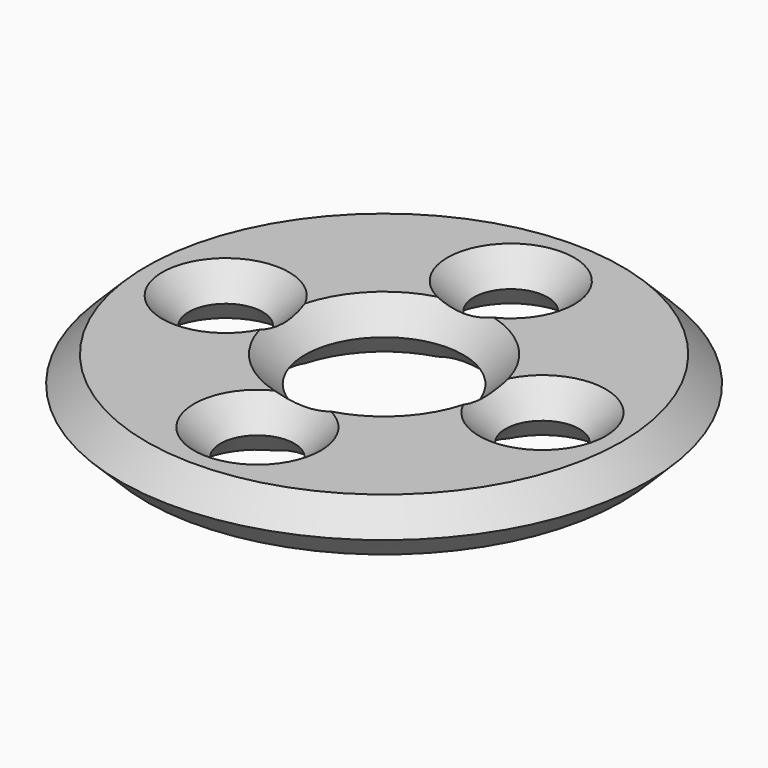
from build123d import *

# Parameters (mm, degrees)
F0_R     = 63.5
F0_R_2   = 19.05
F1_DEPTH = 12.7
F3_D     = 17.78


# Not quite as in the source:
# - a fillet or chamfer that OpenCascade refuses, or shapes differently, is made with other operations: its cross-section is extruded or revolved along the edge and cut away or added


with BuildPart() as f1:
    # F0 (on Top) → F1 (new body)
    with BuildSketch(Plane.XY):
        Circle(F0_R)
        Circle(F0_R_2, mode=Mode.SUBTRACT)
    extrude(amount=F1_DEPTH)

    # F3 (through all)
    with Locations(Plane(origin=(0, 0, 0), x_dir=(1, 0, 0), z_dir=(0, 0, -1))):
        with Locations((0, -38.1), (-38.1, 0), (0, 38.1), (38.1, 0)):
            Hole(F3_D / 2)

    # F4: chamfer of 6.35 on 12 edges, made by hand

    # F4_s1 → F4_t2 (revolve, cut)
    with BuildSketch(Plane.XZ):
        Polygon((25.4, 0), (19.05, 6.35), (19.05, 0), align=None)
    revolve(axis=Axis((0, 0, 0), (0, 0, 1)), mode=Mode.SUBTRACT)

    # F4_s3 → F4_t4 (revolve, cut)
    with BuildSketch(Plane.XZ):
        Polygon((25.4, 12.7), (19.05, 6.35), (19.05, 12.7), align=None)
    revolve(axis=Axis((0, 0, 12.7), (0, 0, 1)), mode=Mode.SUBTRACT)

    # F4_s5 → F4_t6 (revolve, cut)
    with BuildSketch(Plane.XZ):
        Polygon((63.5, 6.35), (57.15, 12.7), (63.5, 12.7), align=None)
    revolve(axis=Axis((0, 0, 12.7), (0, 0, 1)), mode=Mode.SUBTRACT)

    # F4_s7 → F4_t8 (revolve, cut)
    with BuildSketch(Plane.XZ):
        Polygon((63.5, 6.35), (57.15, 0), (63.5, 0), align=None)
    revolve(axis=Axis((0, 0, 0), (0, 0, 1)), mode=Mode.SUBTRACT)

    # F4_s9 → F4_t10 (revolve, cut)
    with BuildSketch(Plane.XZ.offset(38.1)):
        Polygon((15.24, 0), (8.89, 6.35), (8.89, 0), align=None)
    revolve(axis=Axis((0, -38.1, 0), (0, 0, -1)), mode=Mode.SUBTRACT)

    # F4_s11 → F4_t12 (revolve, cut)
    with BuildSketch(Plane.XZ):
        Polygon((-22.86, 0), (-29.21, 6.35), (-29.21, 0), align=None)
    revolve(axis=Axis((-38.1, 0, 0), (0, 0, -1)), mode=Mode.SUBTRACT)

    # F4_s13 → F4_t14 (revolve, cut)
    with BuildSketch(Plane.XZ):
        Polygon((53.34, 0), (46.99, 6.35), (46.99, 0), align=None)
    revolve(axis=Axis((38.1, 0, 0), (0, 0, -1)), mode=Mode.SUBTRACT)

    # F4_s15 → F4_t16 (revolve, cut)
    with BuildSketch(Plane.XZ.offset(-38.1)):
        Polygon((15.24, 0), (8.89, 6.35), (8.89, 0), align=None)
    revolve(axis=Axis((0, 38.1, 0), (0, 0, -1)), mode=Mode.SUBTRACT)

    # F4_s17 → F4_t18 (revolve, cut)
    with BuildSketch(Plane.XZ.offset(38.1)):
        Polygon((15.24, 12.7), (8.89, 6.35), (8.89, 12.7), align=None)
    revolve(axis=Axis((0, -38.1, 12.7), (0, 0, -1)), mode=Mode.SUBTRACT)

    # F4_s19 → F4_t20 (revolve, cut)
    with BuildSketch(Plane.XZ):
        Polygon((-22.86, 12.7), (-29.21, 6.35), (-29.21, 12.7), align=None)
    revolve(axis=Axis((-38.1, 0, 12.7), (0, 0, -1)), mode=Mode.SUBTRACT)

    # F4_s21 → F4_t22 (revolve, cut)
    with BuildSketch(Plane.XZ):
        Polygon((53.34, 12.7), (46.99, 6.35), (46.99, 12.7), align=None)
    revolve(axis=Axis((38.1, 0, 12.7), (0, 0, -1)), mode=Mode.SUBTRACT)

    # F4_s23 → F4_t24 (revolve, cut)
    with BuildSketch(Plane.XZ.offset(-38.1)):
        Polygon((15.24, 12.7), (8.89, 6.35), (8.89, 12.7), align=None)
    revolve(axis=Axis((0, 38.1, 12.7), (0, 0, -1)), mode=Mode.SUBTRACT)


solid = f1.part
